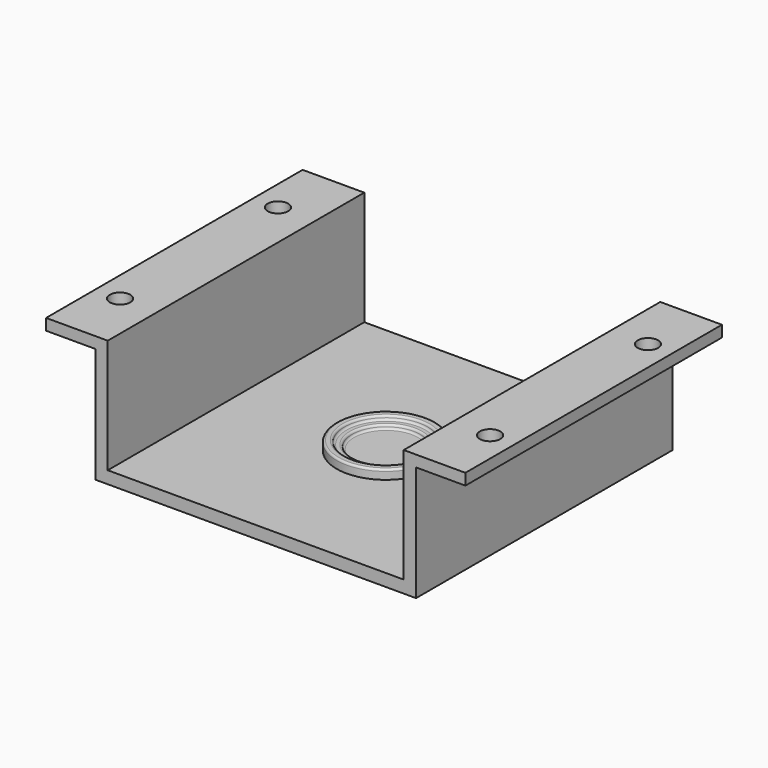
from build123d import *

# Parameters (mm, degrees)
F1_DEPTH = 39
F2_R     = 2.5
F3_DEPTH = 2.748386896
F4_R     = 12.0181970212
F5_DEPTH = 5.3
F6_R     = 10.1005312929
F7_DEPTH = 1
F8_R     = 8.272494484
F9_DEPTH = 1
F10_R    = 0.49999


# Not quite as in the source:
# - a fillet or chamfer is up to 0.001 mm smaller than in the source, because OpenCascade refuses the exact size


with BuildPart() as f1:
    # F0 (on Front) → F1 (new body, symmetric)
    with BuildSketch(Plane.XZ):
        Polygon((33.0240737289, -6.6249261405), (-2.9748248395, -6.6249261405), (-2.9748248395, -9.6249261405), (36.0251751605, -9.6249261405), (36.0251751605, 18.3750738595), (48.0240737289, 18.3750738595), (48.0240737289, 21.1234607555), (33.0240737289, 21.1234607555), align=None)
        Polygon((-2.9748248395, -9.6249261405), (-2.9748248395, -6.6249261405), (-38.9737234078, -6.6249261405), (-38.9737234078, 21.1234607555), (-53.9737234078, 21.1234607555), (-53.9737234078, 18.3750738595), (-41.9748248395, 18.3750738595), (-41.9748248395, -9.6249261405), align=None)
    extrude(amount=F1_DEPTH, both=True)

    # F2 (on face) → F3 (cut, through all)
    with BuildSketch(Plane.XY.offset(21.1234607555)):
        with Locations((42.0246244447, -24)):
            Circle(F2_R)
        with Locations((42.0246244447, 24)):
            Circle(F2_R)
        with Locations((-47.9742741236, 24)):
            Circle(F2_R)
        with Locations((-47.9742741236, -24)):
            Circle(F2_R)
    extrude(amount=-F3_DEPTH, mode=Mode.SUBTRACT)

    # F4 (on face) → F5 (join)
    with BuildSketch(Plane(origin=(0, 0, -9.6249261405), x_dir=(1, 0, 0), z_dir=(0, 0, -1))):
        with Locations((-2.7290005237, -0.3212007869)):
            Circle(F4_R)
    extrude(amount=-F5_DEPTH)

    # F6 (on face) → F7 (cut)
    with BuildSketch(Plane.XY.offset(-4.3249261405)):
        with Locations((-2.7290005237, 0.3212007869)):
            Circle(F6_R)
    extrude(amount=-F7_DEPTH, mode=Mode.SUBTRACT)

    # F8 (on face) → F9 (cut)
    with BuildSketch(Plane.XY.offset(-5.3249261405)):
        with Locations((-2.7290005237, 0.3212007869)):
            Circle(F8_R)
    extrude(amount=-F9_DEPTH, mode=Mode.SUBTRACT)

    # F10 (radius 0.5 in the source; OpenCascade refuses exactly that, so slightly less here)
    f10_edges = [f1.edges().sort_by_distance(p)[0] for p in [
        (-14.747198, 0.321201, -4.324926),
        (-12.829532, 0.321201, -4.324926),
        (-12.829532, 0.321201, -5.324926),
        (-11.001495, 0.321201, -5.324926),
        (-11.001495, 0.321201, -6.324926),
    ]]
    fillet(f10_edges, radius=F10_R)


solid = f1.part
